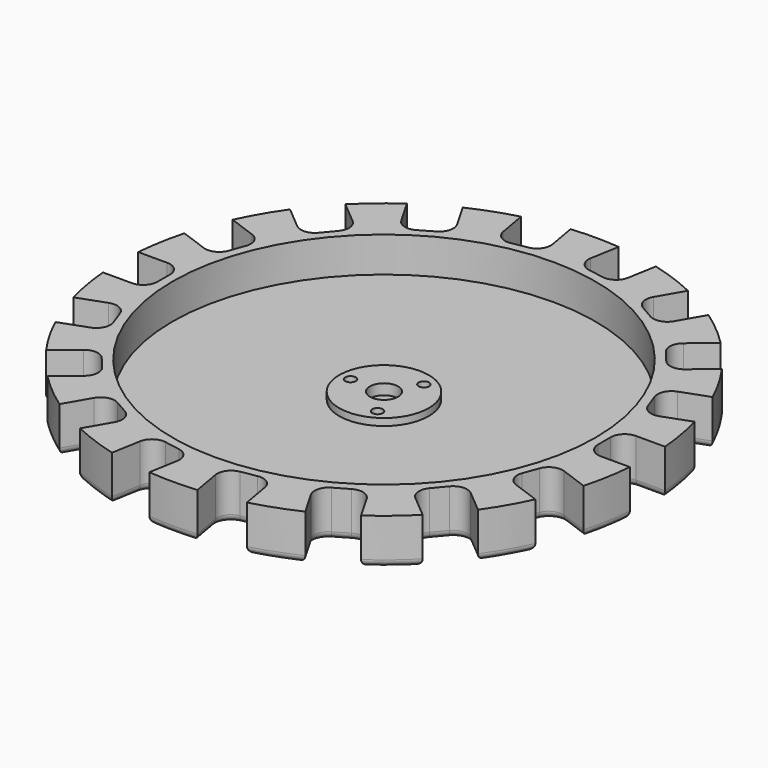
from build123d import *

# Parameters (mm, degrees)
F0_R         = 60
F0_R_2       = 12.7
F0_R_3       = 1.5
F0_R_4       = 4
F1_DEPTH     = 3
F2_DEPTH     = 13
F3_DEPTH     = 5
F4_DEPTH     = 2
F5_R         = 2
F6_TEXT_SIZE = 22.7682912676
F7_DEPTH     = 1


# Not quite as in the source:
# - Text() gives the source's letters only with a copy of the font that has no kerning and outlines rounded to 1/6400 em; it was checked with that copy


with BuildPart() as f1:
    # F0 (on Top) → F1 (new body)
    with BuildSketch(Plane.XY):
        Circle(F0_R)
        Circle(F0_R_2, mode=Mode.SUBTRACT)
        Circle(F0_R_2)
        with Locations((-4.75, -8.227241336)):
            Circle(F0_R_3, mode=Mode.SUBTRACT)
        with Locations((4.75, -8.227241336)):
            Circle(F0_R_3, mode=Mode.SUBTRACT)
        with Locations((-9.5, 0)):
            Circle(F0_R_3, mode=Mode.SUBTRACT)
        with Locations((-4.75, 8.227241336)):
            Circle(F0_R_3, mode=Mode.SUBTRACT)
        Circle(F0_R_4, mode=Mode.SUBTRACT)
        with Locations((4.75, 8.227241336)):
            Circle(F0_R_3, mode=Mode.SUBTRACT)
        with Locations((9.5, 0)):
            Circle(F0_R_3, mode=Mode.SUBTRACT)
        with Locations((9.5, 0)):
            Circle(F0_R_3)
        with Locations((4.75, 8.227241336)):
            Circle(F0_R_3)
        with Locations((-4.75, 8.227241336)):
            Circle(F0_R_3)
        with Locations((-9.5, 0)):
            Circle(F0_R_3)
        with Locations((-4.75, -8.227241336)):
            Circle(F0_R_3)
        with Locations((4.75, -8.227241336)):
            Circle(F0_R_3)
    extrude(amount=F1_DEPTH)

    # F0 (on Top) → F2 (join)
    with BuildSketch(Plane.XY):
        with BuildLine():
            Line((66.5, 6.25), (74.7391296444, 6.25))
            ThreePointArc((74.7391296444, 6.25), (73.8605814759, 13.023613325), (72.3694345066, 19.6892089531))
            Line((72.3694345066, 19.6892089531), (64.627185178, 16.8712606512))
            ThreePointArc((64.627185178, 16.8712606512), (61.5686315578, 17.0047999862), (59.5003341216, 19.2619505611))
            Line((59.5003341216, 19.2619505611), (57.9612434766, 23.4905673546))
            ThreePointArc((57.9612434766, 23.4905673546), (58.0947828116, 26.5491209749), (60.3519333865, 28.6174184111))
            Line((60.3519333865, 28.6174184111), (68.094182715, 31.4353667129))
            ThreePointArc((68.094182715, 31.4353667129), (64.9519052838, 37.5), (61.2709175082, 43.2536087247))
            Line((61.2709175082, 43.2536087247), (54.959378028, 37.9575982747))
            ThreePointArc((54.959378028, 37.9575982747), (52.0396046182, 37.0369972548), (49.3240498167, 38.4506256084))
            Line((49.3240498167, 38.4506256084), (46.4315055731, 41.8978256024))
            ThreePointArc((46.4315055731, 41.8978256024), (45.5109045533, 44.8175990122), (46.9245329069, 47.5331538136))
            Line((46.9245329069, 47.5331538136), (53.2360723871, 52.8291642637))
            ThreePointArc((53.2360723871, 52.8291642637), (48.2090707265, 57.4533332339), (42.7822235958, 61.6009849288))
            Line((42.7822235958, 61.6009849288), (38.6626587737, 54.4656893517))
            ThreePointArc((38.6626587737, 54.4656893517), (36.2338333389, 52.6019860465), (33.1985571585, 53.0015877365))
            Line((33.1985571585, 53.0015877365), (29.3014428415, 55.2515877365))
            ThreePointArc((29.3014428415, 55.2515877365), (27.4377395363, 57.6804131713), (27.8373412263, 60.7156893517))
            Line((27.8373412263, 60.7156893517), (31.9569060485, 67.8509849288))
            ThreePointArc((31.9569060485, 67.8509849288), (25.6515107494, 70.4769465589), (19.1333621195, 72.5183732168))
            Line((19.1333621195, 72.5183732168), (17.7026522712, 64.4044144649))
            ThreePointArc((17.7026522712, 64.4044144649), (16.0577270045, 61.8223989984), (13.0688285485, 61.1597761635))
            Line((13.0688285485, 61.1597761635), (8.6371936599, 61.941192963))
            ThreePointArc((8.6371936599, 61.941192963), (6.0551781934, 63.5861182297), (5.3925553585, 66.5750166857))
            Line((5.3925553585, 66.5750166857), (6.8232652068, 74.6889754376))
            ThreePointArc((6.8232652068, 74.6889754376), (0, 75), (-6.8232652068, 74.6889754376))
            Line((-6.8232652068, 74.6889754376), (-5.3925553585, 66.5750166857))
            ThreePointArc((-5.3925553585, 66.5750166857), (-6.0551781934, 63.5861182297), (-8.6371936599, 61.941192963))
            Line((-8.6371936599, 61.941192963), (-13.0688285485, 61.1597761635))
            ThreePointArc((-13.0688285485, 61.1597761635), (-16.0577270045, 61.8223989984), (-17.7026522712, 64.4044144649))
            Line((-17.7026522712, 64.4044144649), (-19.1333621195, 72.5183732168))
            ThreePointArc((-19.1333621195, 72.5183732168), (-25.6515107494, 70.4769465589), (-31.9569060485, 67.8509849288))
            Line((-31.9569060485, 67.8509849288), (-27.8373412263, 60.7156893517))
            ThreePointArc((-27.8373412263, 60.7156893517), (-27.4377395363, 57.6804131713), (-29.3014428415, 55.2515877365))
            Line((-29.3014428415, 55.2515877365), (-33.1985571585, 53.0015877365))
            ThreePointArc((-33.1985571585, 53.0015877365), (-36.2338333389, 52.6019860465), (-38.6626587737, 54.4656893517))
            Line((-38.6626587737, 54.4656893517), (-42.7822235958, 61.6009849288))
            ThreePointArc((-42.7822235958, 61.6009849288), (-48.2090707265, 57.4533332339), (-53.2360723871, 52.8291642637))
            Line((-53.2360723871, 52.8291642637), (-46.9245329069, 47.5331538136))
            ThreePointArc((-46.9245329069, 47.5331538136), (-45.5109045533, 44.8175990122), (-46.4315055731, 41.8978256024))
            Line((-46.4315055731, 41.8978256024), (-49.3240498167, 38.4506256084))
            ThreePointArc((-49.3240498167, 38.4506256084), (-52.0396046182, 37.0369972548), (-54.959378028, 37.9575982747))
            Line((-54.959378028, 37.9575982747), (-61.2709175082, 43.2536087247))
            ThreePointArc((-61.2709175082, 43.2536087247), (-64.9519052838, 37.5), (-68.094182715, 31.4353667129))
            Line((-68.094182715, 31.4353667129), (-60.3519333865, 28.6174184111))
            ThreePointArc((-60.3519333865, 28.6174184111), (-58.0947828116, 26.5491209749), (-57.9612434766, 23.4905673546))
            Line((-57.9612434766, 23.4905673546), (-59.5003341216, 19.2619505611))
            ThreePointArc((-59.5003341216, 19.2619505611), (-61.5686315578, 17.0047999862), (-64.627185178, 16.8712606512))
            Line((-64.627185178, 16.8712606512), (-72.3694345066, 19.6892089531))
            ThreePointArc((-72.3694345066, 19.6892089531), (-73.8605814759, 13.023613325), (-74.7391296444, 6.25))
            Line((-74.7391296444, 6.25), (-66.5, 6.25))
            ThreePointArc((-66.5, 6.25), (-63.6715728753, 5.0784271247), (-62.5, 2.25))
            Line((-62.5, 2.25), (-62.5, -2.25))
            ThreePointArc((-62.5, -2.25), (-63.6715728753, -5.0784271247), (-66.5, -6.25))
            Line((-66.5, -6.25), (-74.7391296444, -6.25))
            ThreePointArc((-74.7391296444, -6.25), (-73.8605814759, -13.023613325), (-72.3694345066, -19.6892089531))
            Line((-72.3694345066, -19.6892089531), (-64.627185178, -16.8712606512))
            ThreePointArc((-64.627185178, -16.8712606512), (-61.5686315578, -17.0047999862), (-59.5003341216, -19.2619505611))
            Line((-59.5003341216, -19.2619505611), (-57.9612434766, -23.4905673546))
            ThreePointArc((-57.9612434766, -23.4905673546), (-58.0947828116, -26.5491209749), (-60.3519333865, -28.6174184111))
            Line((-60.3519333865, -28.6174184111), (-68.094182715, -31.4353667129))
            ThreePointArc((-68.094182715, -31.4353667129), (-64.9519052838, -37.5), (-61.2709175082, -43.2536087247))
            Line((-61.2709175082, -43.2536087247), (-54.959378028, -37.9575982747))
            ThreePointArc((-54.959378028, -37.9575982747), (-52.0396046182, -37.0369972548), (-49.3240498167, -38.4506256084))
            Line((-49.3240498167, -38.4506256084), (-46.4315055731, -41.8978256024))
            ThreePointArc((-46.4315055731, -41.8978256024), (-45.5109045533, -44.8175990122), (-46.9245329069, -47.5331538136))
            Line((-46.9245329069, -47.5331538136), (-53.2360723871, -52.8291642637))
            ThreePointArc((-53.2360723871, -52.8291642637), (-48.2090707265, -57.4533332339), (-42.7822235958, -61.6009849288))
            Line((-42.7822235958, -61.6009849288), (-38.6626587737, -54.4656893517))
            ThreePointArc((-38.6626587737, -54.4656893517), (-36.2338333389, -52.6019860465), (-33.1985571585, -53.0015877365))
            Line((-33.1985571585, -53.0015877365), (-29.3014428415, -55.2515877365))
            ThreePointArc((-29.3014428415, -55.2515877365), (-27.4377395363, -57.6804131713), (-27.8373412263, -60.7156893517))
            Line((-27.8373412263, -60.7156893517), (-31.9569060485, -67.8509849288))
            ThreePointArc((-31.9569060485, -67.8509849288), (-25.6515107494, -70.4769465589), (-19.1333621195, -72.5183732168))
            Line((-19.1333621195, -72.5183732168), (-17.7026522712, -64.4044144649))
            ThreePointArc((-17.7026522712, -64.4044144649), (-16.0577270045, -61.8223989984), (-13.0688285485, -61.1597761635))
            Line((-13.0688285485, -61.1597761635), (-8.6371936599, -61.941192963))
            ThreePointArc((-8.6371936599, -61.941192963), (-6.0551781934, -63.5861182297), (-5.3925553585, -66.5750166857))
            Line((-5.3925553585, -66.5750166857), (-6.8232652068, -74.6889754376))
            ThreePointArc((-6.8232652068, -74.6889754376), (0, -75), (6.8232652068, -74.6889754376))
            Line((6.8232652068, -74.6889754376), (5.3925553585, -66.5750166857))
            ThreePointArc((5.3925553585, -66.5750166857), (6.0551781934, -63.5861182297), (8.6371936599, -61.941192963))
            Line((8.6371936599, -61.941192963), (13.0688285485, -61.1597761635))
            ThreePointArc((13.0688285485, -61.1597761635), (16.0577270045, -61.8223989984), (17.7026522712, -64.4044144649))
            Line((17.7026522712, -64.4044144649), (19.1333621195, -72.5183732168))
            ThreePointArc((19.1333621195, -72.5183732168), (25.6515107494, -70.4769465589), (31.9569060485, -67.8509849288))
            Line((31.9569060485, -67.8509849288), (27.8373412263, -60.7156893517))
            ThreePointArc((27.8373412263, -60.7156893517), (27.4377395363, -57.6804131713), (29.3014428415, -55.2515877365))
            Line((29.3014428415, -55.2515877365), (33.1985571585, -53.0015877365))
            ThreePointArc((33.1985571585, -53.0015877365), (36.2338333389, -52.6019860465), (38.6626587737, -54.4656893517))
            Line((38.6626587737, -54.4656893517), (42.7822235958, -61.6009849288))
            ThreePointArc((42.7822235958, -61.6009849288), (48.2090707265, -57.4533332339), (53.2360723871, -52.8291642637))
            Line((53.2360723871, -52.8291642637), (46.9245329069, -47.5331538136))
            ThreePointArc((46.9245329069, -47.5331538136), (45.5109045533, -44.8175990122), (46.4315055731, -41.8978256024))
            Line((46.4315055731, -41.8978256024), (49.3240498167, -38.4506256084))
            ThreePointArc((49.3240498167, -38.4506256084), (52.0396046182, -37.0369972548), (54.959378028, -37.9575982747))
            Line((54.959378028, -37.9575982747), (61.2709175082, -43.2536087247))
            ThreePointArc((61.2709175082, -43.2536087247), (64.9519052838, -37.5), (68.094182715, -31.4353667129))
            Line((68.094182715, -31.4353667129), (60.3519333865, -28.6174184111))
            ThreePointArc((60.3519333865, -28.6174184111), (58.0947828116, -26.5491209749), (57.9612434766, -23.4905673546))
            Line((57.9612434766, -23.4905673546), (59.5003341216, -19.2619505611))
            ThreePointArc((59.5003341216, -19.2619505611), (61.5686315578, -17.0047999862), (64.627185178, -16.8712606512))
            Line((64.627185178, -16.8712606512), (72.3694345066, -19.6892089531))
            ThreePointArc((72.3694345066, -19.6892089531), (73.8605814759, -13.023613325), (74.7391296444, -6.25))
            Line((74.7391296444, -6.25), (66.5, -6.25))
            ThreePointArc((66.5, -6.25), (63.6715728753, -5.0784271247), (62.5, -2.25))
            Line((62.5, -2.25), (62.5, 2.25))
            ThreePointArc((62.5, 2.25), (63.6715728753, 5.0784271247), (66.5, 6.25))
        make_face()
        Circle(F0_R, mode=Mode.SUBTRACT)
    extrude(amount=F2_DEPTH)

    # F0 (on Top) → F3 (join)
    with BuildSketch(Plane.XY):
        Circle(F0_R_2)
        with Locations((-4.75, -8.227241336)):
            Circle(F0_R_3, mode=Mode.SUBTRACT)
        with Locations((4.75, -8.227241336)):
            Circle(F0_R_3, mode=Mode.SUBTRACT)
        with Locations((-9.5, 0)):
            Circle(F0_R_3, mode=Mode.SUBTRACT)
        with Locations((-4.75, 8.227241336)):
            Circle(F0_R_3, mode=Mode.SUBTRACT)
        Circle(F0_R_4, mode=Mode.SUBTRACT)
        with Locations((4.75, 8.227241336)):
            Circle(F0_R_3, mode=Mode.SUBTRACT)
        with Locations((9.5, 0)):
            Circle(F0_R_3, mode=Mode.SUBTRACT)
        with Locations((-4.75, 8.227241336)):
            Circle(F0_R_3)
        with Locations((9.5, 0)):
            Circle(F0_R_3)
        with Locations((-4.75, -8.227241336)):
            Circle(F0_R_3)
    extrude(amount=F3_DEPTH)

    # F0 (on Top) → F4 (join)
    with BuildSketch(Plane.XY):
        Circle(F0_R_4)
    extrude(amount=F4_DEPTH)

    # F5
    f5_edges = [f1.edges().sort_by_distance(p)[0] for p in [
        (50.080303, -50.181159, 0),
        (45.510905, -44.817599, 0),
        (47.877778, -40.174226, 0),
        (52.039605, -37.036997, 0),
        (58.115148, -40.605603, 0),
        (64.951905, -37.5, 0),
        (64.223058, -30.026393, 0),
        (58.094783, -26.549121, 0),
        (58.730789, -21.376259, 0),
        (61.568632, -17.0048, 0),
        (68.49831, -18.280235, 0),
        (73.860581, -13.023613, 0),
        (70.619565, -6.25, 0),
        (63.671573, -5.078427, 0),
        (62.5, 0, 0),
        (63.671573, 5.078427, 0),
        (70.619565, 6.25, 0),
        (73.860581, 13.023613, 0),
        (68.49831, 18.280235, 0),
        (61.568632, 17.0048, 0),
        (58.730789, 21.376259, 0),
        (58.094783, 26.549121, 0),
        (64.223058, 30.026393, 0),
        (64.951905, 37.5, 0),
        (58.115148, 40.605603, 0),
        (52.039605, 37.036997, 0),
        (47.877778, 40.174226, 0),
        (45.510905, 44.817599, 0),
        (50.080303, 50.181159, 0),
        (48.209071, 57.453333, 0),
        (40.722441, 58.033337, 0),
        (36.233833, 52.601986, 0),
        (31.25, 54.126588, 0),
        (27.43774, 57.680413, 0),
        (29.897124, 64.283337, 0),
        (25.651511, 70.476947, 0),
        (18.418007, 68.461394, 0),
        (16.057727, 61.822399, 0),
        (10.853011, 61.550485, 0),
        (6.055178, 63.586118, 0),
        (6.10791, 70.631996, 0),
        (0, 75, 0),
        (-6.10791, 70.631996, 0),
        (-6.055178, 63.586118, 0),
        (-10.853011, 61.550485, 0),
        (-16.057727, 61.822399, 0),
        (-18.418007, 68.461394, 0),
        (-25.651511, 70.476947, 0),
        (-29.897124, 64.283337, 0),
        (-27.43774, 57.680413, 0),
        (-31.25, 54.126588, 0),
        (-36.233833, 52.601986, 0),
        (-40.722441, 58.033337, 0),
        (-48.209071, 57.453333, 0),
        (-50.080303, 50.181159, 0),
        (-45.510905, 44.817599, 0),
        (-47.877778, 40.174226, 0),
        (-52.039605, 37.036997, 0),
        (-58.115148, 40.605603, 0),
        (-64.951905, 37.5, 0),
        (-64.223058, 30.026393, 0),
        (-58.094783, 26.549121, 0),
        (-58.730789, 21.376259, 0),
        (-61.568632, 17.0048, 0),
        (-68.49831, 18.280235, 0),
        (-73.860581, 13.023613, 0),
        (-70.619565, 6.25, 0),
        (-63.671573, 5.078427, 0),
        (-62.5, 0, 0),
        (-63.671573, -5.078427, 0),
        (-70.619565, -6.25, 0),
        (-73.860581, -13.023613, 0),
        (-68.49831, -18.280235, 0),
        (-61.568632, -17.0048, 0),
        (-58.730789, -21.376259, 0),
        (-58.094783, -26.549121, 0),
        (-64.223058, -30.026393, 0),
        (-64.951905, -37.5, 0),
        (-58.115148, -40.605603, 0),
        (-52.039605, -37.036997, 0),
        (-47.877778, -40.174226, 0),
        (-45.510905, -44.817599, 0),
        (-50.080303, -50.181159, 0),
        (-48.209071, -57.453333, 0),
        (-40.722441, -58.033337, 0),
        (-36.233833, -52.601986, 0),
        (-31.25, -54.126588, 0),
        (-27.43774, -57.680413, 0),
        (-29.897124, -64.283337, 0),
        (-25.651511, -70.476947, 0),
        (-18.418007, -68.461394, 0),
        (-16.057727, -61.822399, 0),
        (-10.853011, -61.550485, 0),
        (-6.055178, -63.586118, 0),
        (-6.10791, -70.631996, 0),
        (0, -75, 0),
        (6.10791, -70.631996, 0),
        (6.055178, -63.586118, 0),
        (10.853011, -61.550485, 0),
        (16.057727, -61.822399, 0),
        (18.418007, -68.461394, 0),
        (25.651511, -70.476947, 0),
        (29.897124, -64.283337, 0),
        (27.43774, -57.680413, 0),
        (31.25, -54.126588, 0),
        (36.233833, -52.601986, 0),
        (40.722441, -58.033337, 0),
        (48.209071, -57.453333, 0),
    ]]
    fillet(f5_edges, radius=F5_R)

    # F6 (on face) → F7 (cut)
    with BuildSketch(Plane(origin=(0, 0, 0), x_dir=(1, 0, 0), z_dir=(0, 0, -1))):
        with Locations((-41.1132488362, 16.5496473273)):
            Text('.45 ACP', F6_TEXT_SIZE, font='Open Sans', font_style=FontStyle.BOLD, text_align=(TextAlign.LEFT, TextAlign.BOTTOM))
    extrude(amount=-F7_DEPTH, mode=Mode.SUBTRACT)


solid = f1.part
